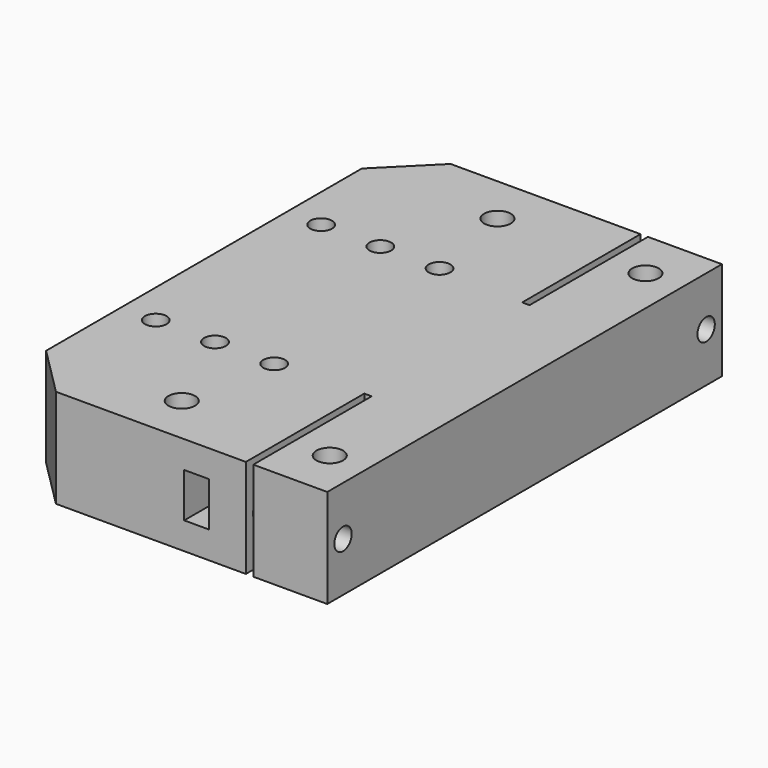
from build123d import *

# Parameters (mm, degrees)
F0_W      = 45
F0_H      = 100
F0_R      = 2.7
F1_DEPTH  = 20
F2_W      = 1.5
F2_H      = 30
F3_DEPTH  = 25
F4_R      = 2.2
F5_DEPTH  = 25
F6_DEPTH  = 20
F7_R      = 5.2
F8_DEPTH  = 40
F9_W      = 2
F9_H      = 9
F10_DEPTH = 40
F11_W     = 2
F11_H     = 15
F12_DEPTH = 10
F13_R     = 2.2
F14_DEPTH = 25
F15_SIZE  = 10
F16_W     = 5
F16_H     = 9
F17_DEPTH = 10


# Not quite as in the source:
# - a pattern or mirror of a feature is missing from the dataset's text; its kind, count and spacing are read off the source's solid


with BuildPart() as f1:
    # F0 (on Top) → F1 (new body)
    with BuildSketch(Plane.XY):
        Rectangle(F0_W, F0_H)
        with Locations((-15, -40)):
            Circle(F0_R, mode=Mode.SUBTRACT)
        with Locations((15, -40)):
            Circle(F0_R, mode=Mode.SUBTRACT)
        with Locations((-15, 40)):
            Circle(F0_R, mode=Mode.SUBTRACT)
        with Locations((15, 40)):
            Circle(F0_R, mode=Mode.SUBTRACT)
    extrude(amount=F1_DEPTH)

    # F2 (on face) → F3 (cut)
    with BuildSketch(Plane.XY.offset(20)):
        with Locations((6.75, -35)):
            Rectangle(F2_W, F2_H)
    f3 = extrude(amount=-F3_DEPTH, mode=Mode.SUBTRACT)

    # F3_copies: F3 across plane
    add(f3.mirror(Plane.ZX), mode=Mode.SUBTRACT)

    # F4 (on face) → F5 (cut)
    with BuildSketch(Plane.YZ.offset(22.5)):
        with Locations((-46, 10)):
            Circle(F4_R)
    f5 = extrude(amount=-F5_DEPTH, mode=Mode.SUBTRACT)

    # F5_copies: F5 across plane
    add(f5.mirror(Plane.ZX), mode=Mode.SUBTRACT)

    # F6 (add): a face of the model
    f6_faces = [f1.faces().sort_by_distance(p)[0] for p in [
        (-22.5, 0, 10),
    ]]
    extrude(f6_faces, amount=F6_DEPTH)

    # F7 (on face) → F8 (cut)
    with BuildSketch(Plane(origin=(-42.5, 0, 0), x_dir=(0, -1, 0), z_dir=(-1, 0, 0))):
        with Locations((-30, 10)):
            Circle(F7_R)
        with Locations((30, 10)):
            Circle(F7_R)
    extrude(amount=-F8_DEPTH, mode=Mode.SUBTRACT)

    # F9 (on face) → F10 (cut)
    with BuildSketch(Plane(origin=(-42.5, 0, 0), x_dir=(0, -1, 0), z_dir=(-1, 0, 0))):
        with Locations((-16, 4.5)):
            Rectangle(F9_W, F9_H)
        Polygon((-17, 9), (-15, 9), (-15, 11), (-30, 11), (-30, 9), align=None)
    f10 = extrude(amount=-F10_DEPTH, mode=Mode.SUBTRACT)

    # F10_copies: F10 across plane
    add(f10.mirror(Plane(origin=(0, 0, 0), x_dir=(0, 0, -1), z_dir=(0, -1, 0))), mode=Mode.SUBTRACT)

    # F11 (on face) → F12 (cut)
    with BuildSketch(Plane(origin=(0, 0, 0), x_dir=(1, 0, 0), z_dir=(0, 0, -1))):
        with Locations((-3.5, -22.5)):
            Rectangle(F11_W, F11_H)
    f12 = extrude(amount=-F12_DEPTH, mode=Mode.SUBTRACT)

    # F12_copies: F12 across plane
    add(f12.mirror(Plane(origin=(0, 0, 0), x_dir=(0, 0, -1), z_dir=(0, -1, 0))), mode=Mode.SUBTRACT)

    # F13 (on face) → F14 (cut, symmetric)
    with BuildSketch(Plane.XY.offset(9)):
        with Locations((-35.5, 20.9485298356)):
            Circle(F13_R)
        with Locations((-11.5, 20.9485298356)):
            Circle(F13_R)
        with Locations((-23.5, 20.9485298356)):
            Circle(F13_R)
    f14 = extrude(amount=F14_DEPTH, both=True, mode=Mode.SUBTRACT)

    # F14_copies: F14 across plane
    add(f14.mirror(Plane(origin=(0, 0, 0), x_dir=(0, 0, -1), z_dir=(0, -1, 0))), mode=Mode.SUBTRACT)

    # F15
    f15_edges = [f1.edges().sort_by_distance(p)[0] for p in [
        (-42.5, 50, 10),
        (-42.5, -50, 10),
    ]]
    chamfer(f15_edges, length=F15_SIZE)

    # F16 (on face) → F17 (cut)
    with BuildSketch(Plane.XZ.offset(50)):
        with Locations((-4, 10)):
            Rectangle(F16_W, F16_H)
    f17 = extrude(amount=-F17_DEPTH, mode=Mode.SUBTRACT)

    # F17_copies: F17 across plane
    add(f17.mirror(Plane.ZX), mode=Mode.SUBTRACT)


solid = f1.part
